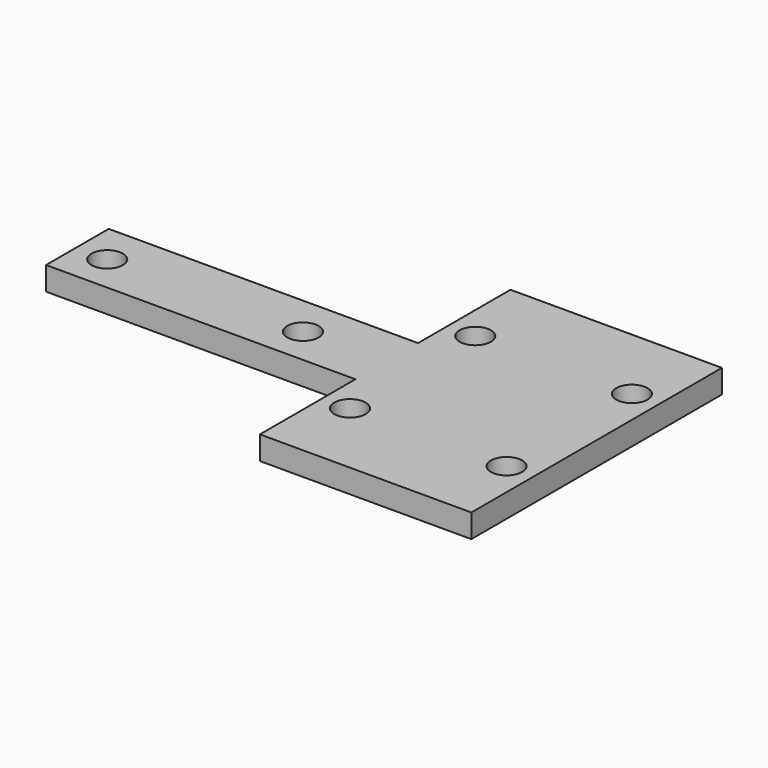
from build123d import *

# Parameters (mm, degrees)
F1_DEPTH = 3
F2_D     = 4


with BuildPart() as f1:
    # F0 (on Top) → F1 (new body)
    with BuildSketch(Plane.XY):
        Polygon((-13.5, -20), (13.5, -20), (13.5, 20), (-13.5, 20), (-13.5, 5.2414399013), (-53, 5.2414399013), (-53, -4.7585600987), (-13.5, -4.7585600987), align=None)
    extrude(amount=F1_DEPTH)

    # F2 (through all)
    with Locations(Plane(origin=(0, 0, 0), x_dir=(1, 0, 0), z_dir=(0, 0, -1))):
        with Locations((-49, 0), (-24, 0), (-10, 10), (10, -10), (10, 10), (-10, -10)):
            Hole(F2_D / 2)


solid = f1.part
